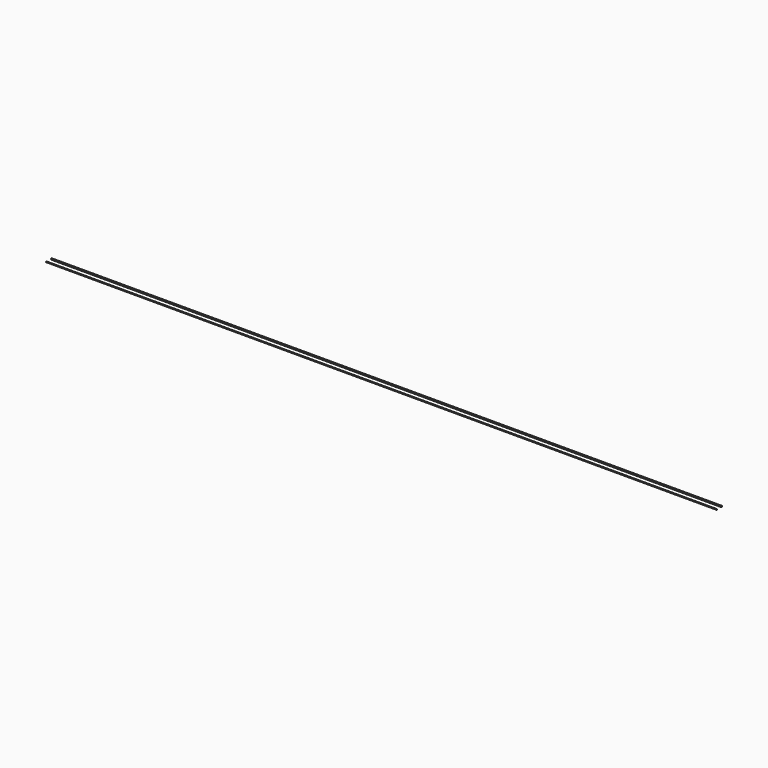
from build123d import *

# Parameters (mm, degrees)
F2_DEPTH = 2000


with BuildPart() as f2:
    # F1 (on Right) → F2 (new body)
    with BuildSketch(Plane.YZ):
        with BuildLine():
            Line((-10, -7.4163670351), (-10, -10))
            Line((-10, -10), (-7.4163670351, -10))
            ThreePointArc((-7.4163670351, -10), (-8.8034794258, -8.8034794258), (-10, -7.4163670351))
        make_face()
    extrude(amount=F2_DEPTH)


with BuildPart() as f2b:
    # F1 (on Right) → F2, piece 2 (new body)
    with BuildSketch(Plane.YZ):
        with BuildLine():
            ThreePointArc((10, -7.4163670351), (8.8034794258, -8.8034794258), (7.4163670351, -10))
            Line((7.4163670351, -10), (10, -10))
            Line((10, -10), (10, -7.4163670351))
        make_face()
    extrude(amount=F2_DEPTH)


solid = Compound([f2.part, f2b.part])
